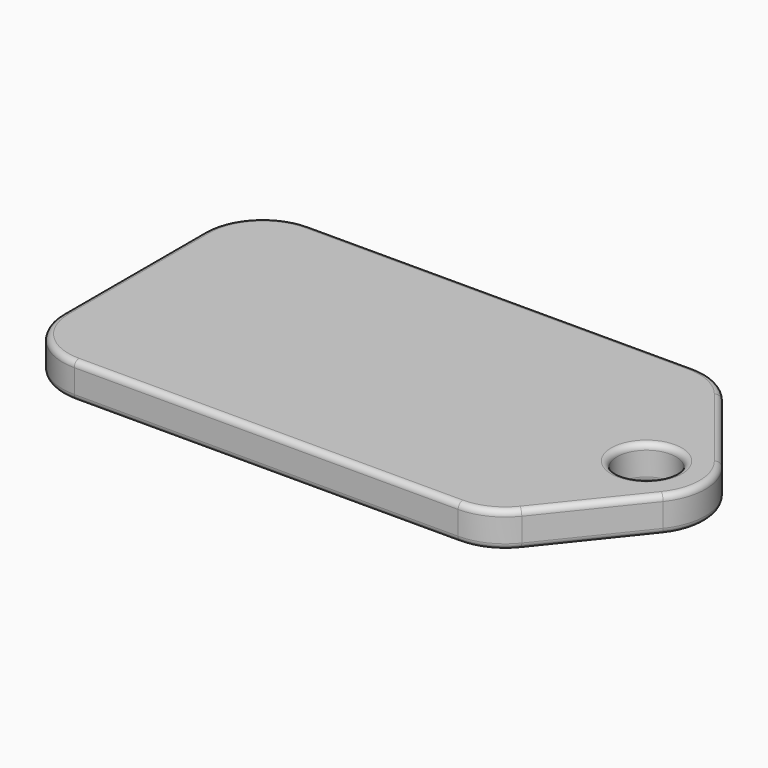
from build123d import *

# Parameters (mm, degrees)
F1_DEPTH     = 3
F2_R         = 5
F4_D         = 5
F5_R         = 5
F6_R         = 0.5
F7_TEXT_SIZE = 15.329418885
F8_DEPTH     = 1


# Not quite as in the source:
# - Text() gives the source's letters only with a copy of the font that has no kerning and outlines rounded to 1/6400 em; it was checked with that copy


with BuildPart() as f1:
    # F0 (on Top) → F1 (new body)
    with BuildSketch(Plane.XY):
        Polygon((20, 12.5), (-20, 12.5), (-20, -12.5), (20, -12.5), (30, 0), align=None)
    extrude(amount=F1_DEPTH)

    # F2
    f2_edges = [f1.edges().sort_by_distance(p)[0] for p in [
        (30, 0, 1.5),
    ]]
    fillet(f2_edges, radius=F2_R)

    # F4 (through all)
    with Locations(Plane.XY.offset(3)):
        with Locations((23.5968757626, 0)):
            Hole(F4_D / 2)

    # F5
    f5_edges = [f1.edges().sort_by_distance(p)[0] for p in [
        (20, 12.5, 1.5),
        (-20, 12.5, 1.5),
        (-20, -12.5, 1.5),
        (20, -12.5, 1.5),
    ]]
    fillet(f5_edges, radius=F5_R)

    # F6
    f6_edges = [f1.edges().sort_by_distance(p)[0] for p in [
        (1.298438, 12.5, 3),
        (24.50122, -6.873475, 0),
        (19.762819, -12.006516, 0),
        (28.596876, 0, 0),
        (1.298438, -12.5, 0),
        (24.50122, 6.873475, 0),
        (-18.535534, -11.035534, 0),
        (19.762819, 12.006516, 0),
        (-20, 0, 0),
        (1.298438, 12.5, 0),
        (-18.535534, 11.035534, 0),
        (21.096876, 0, 0),
        (24.50122, -6.873475, 3),
        (19.762819, -12.006516, 3),
        (28.596876, 0, 3),
        (1.298438, -12.5, 3),
        (24.50122, 6.873475, 3),
        (-18.535534, -11.035534, 3),
        (19.762819, 12.006516, 3),
        (-20, 0, 3),
        (-18.535534, 11.035534, 3),
        (21.096876, 0, 3),
    ]]
    fillet(f6_edges, radius=F6_R)

    # F7 (on face) → F8 (cut)
    with BuildSketch(Plane(origin=(0, 0, 0), x_dir=(1, 0, 0), z_dir=(0, 0, -1))):
        with Locations((-16.1203499883, -5.0893672742)):
            Text('Gary', F7_TEXT_SIZE, font='Open Sans', text_align=(TextAlign.LEFT, TextAlign.BOTTOM))
    extrude(amount=-F8_DEPTH, mode=Mode.SUBTRACT)


solid = f1.part
